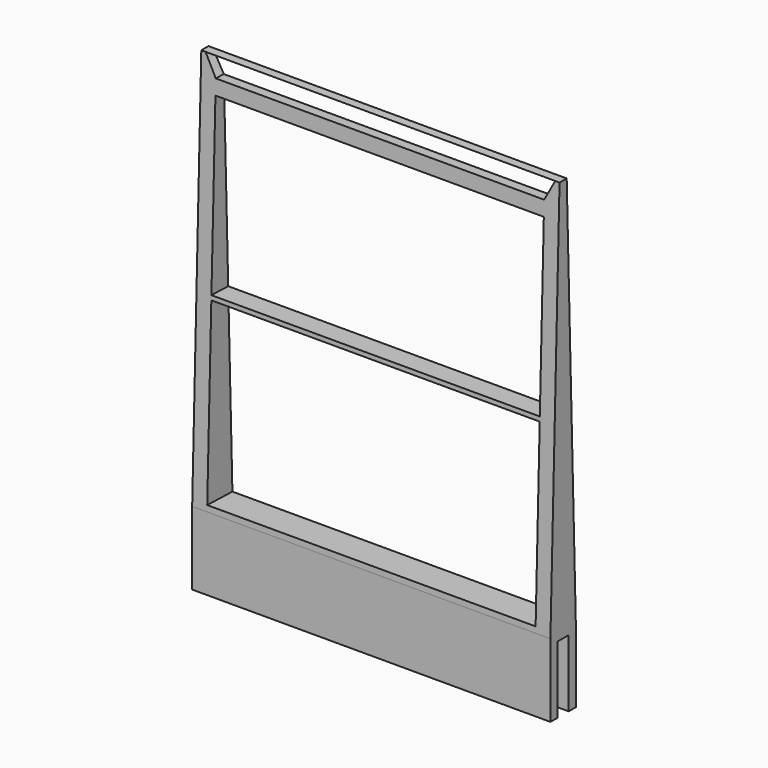
from build123d import *

# Parameters (mm, degrees)
F1_DEPTH = 40
F2_W     = 73.3336731791
F2_H     = 38.809017675
F2_H_2   = 1
F3_DEPTH = 7.5685053212


# Not quite as in the source:
# - a feature names something its author has since deleted; it is built from what else it names


with BuildPart() as f1:
    # F0 (on Right) → F1 (new body, symmetric)
    with BuildSketch(Plane.YZ):
        Polygon((-1.55, -15), (-1.55, 0), (1.55, 0), (1.55, -15), (3.55, -15), (3.55, 1.359729562), (1, 90), (-1, 90), (-3.55, 1.359729562), (-3.55, 0), (-3.55, -15), align=None)
    extrude(amount=F1_DEPTH, both=True)

    # F2 (on face) → F3 (cut, through all)
    with BuildSketch(Plane(origin=(0, -3.5861487682, 0.1031661943), x_dir=(1, 0, 0), z_dir=(0, -0.9995864588, 0.028756066))):
        Polygon((36.6668365896, 85.5283662677), (39.0464413553, 89.9340252282), (-39.0464413553, 89.9340252282), (-36.6668365896, 85.5283662677), align=None)
        with Locations((0, 62.7911531245)):
            Rectangle(F2_W, F2_H)
        with Locations((0, 41.886644287)):
            Rectangle(F2_W, F2_H_2)
        with Locations((0, 21.9821354495)):
            Rectangle(F2_W, F2_H)
    extrude(amount=-F3_DEPTH, mode=Mode.SUBTRACT)


solid = f1.part
